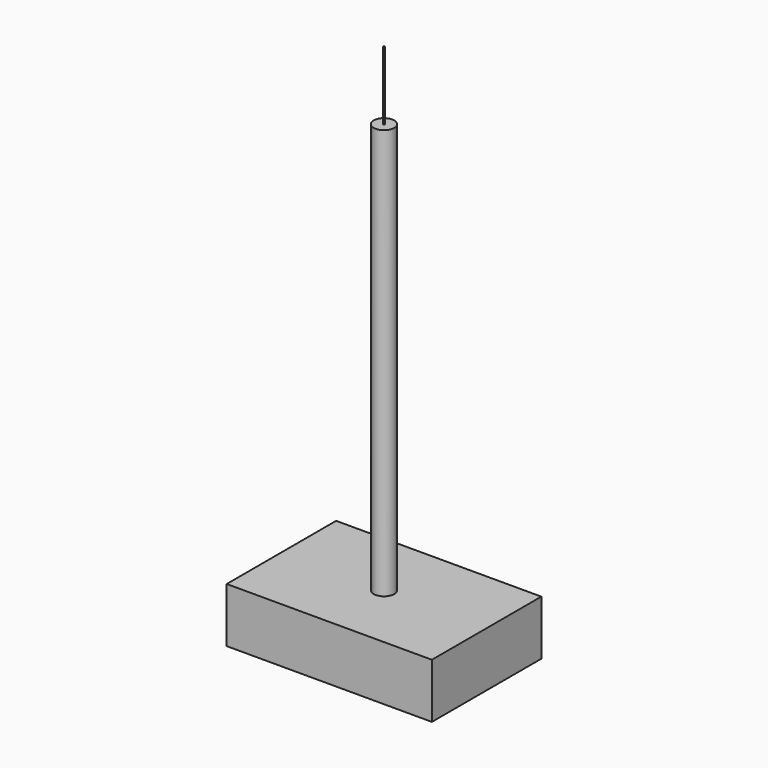
from build123d import *

# Parameters (mm, degrees)
F0_W     = 150
F0_H     = 100
F1_DEPTH = 40
F2_R     = 0.5
F3_DEPTH = 350
F2_R_2   = 7.5
F4_DEPTH = 300


with BuildPart() as f1:
    # F0 (on Top) → F1 (new body)
    with BuildSketch(Plane.XY):
        Rectangle(F0_W, F0_H)
    extrude(amount=-F1_DEPTH)

    # F2 (on Top) → F4 (join)
    with BuildSketch(Plane.XY):
        Circle(F2_R_2)
        Circle(F2_R, mode=Mode.SUBTRACT)
    extrude(amount=F4_DEPTH)


with BuildPart() as f3:
    # F2 (on Top) → F3 (new body)
    with BuildSketch(Plane.XY):
        Circle(F2_R)
    extrude(amount=F3_DEPTH)


solid = Compound([f1.part, f3.part])
